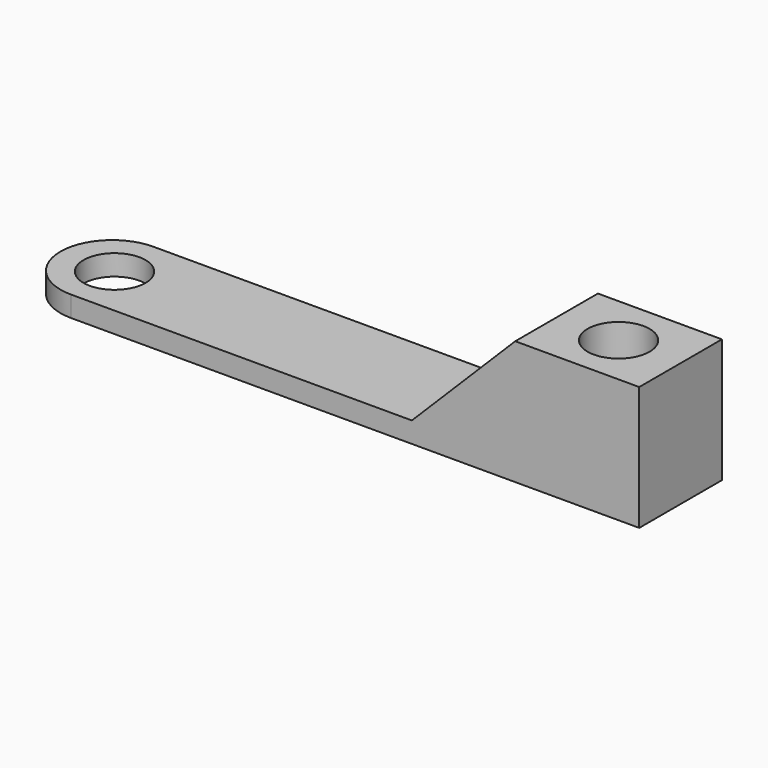
from build123d import *

# Parameters (mm, degrees)
F1_DEPTH = 12.5
F2_R     = 7.5
F3_DEPTH = 30
F5_R     = 12.49999
F4_R     = 7.5
F6_DEPTH = 5


# Not quite as in the source:
# - a fillet or chamfer is up to 0.001 mm smaller than in the source, because OpenCascade refuses the exact size


with BuildPart() as f1:
    # F0 (on Front) → F1 (new body, symmetric)
    with BuildSketch(Plane.XZ):
        Polygon((-150, 0), (0, 0), (0, 30), (-30, 30), (-55, 5), (-150, 5), align=None)
    extrude(amount=F1_DEPTH, both=True)

    # F2 (on face) → F3 (cut, through all)
    with BuildSketch(Plane.XY.offset(30)):
        with Locations((-15, 0)):
            Circle(F2_R)
    extrude(amount=-F3_DEPTH, mode=Mode.SUBTRACT)

    # F5 (radius 12.5 in the source; OpenCascade refuses exactly that, so slightly less here)
    f5_edges = [f1.edges().sort_by_distance(p)[0] for p in [
        (-150, 12.5, 2.5),
        (-150, -12.5, 2.5),
    ]]
    fillet(f5_edges, radius=F5_R)

    # F4 (on face) → F6 (cut, through all)
    with BuildSketch(Plane.XY.offset(5)):
        with Locations((-136.9243115187, 0)):
            Circle(F4_R)
    extrude(amount=-F6_DEPTH, mode=Mode.SUBTRACT)


solid = f1.part
